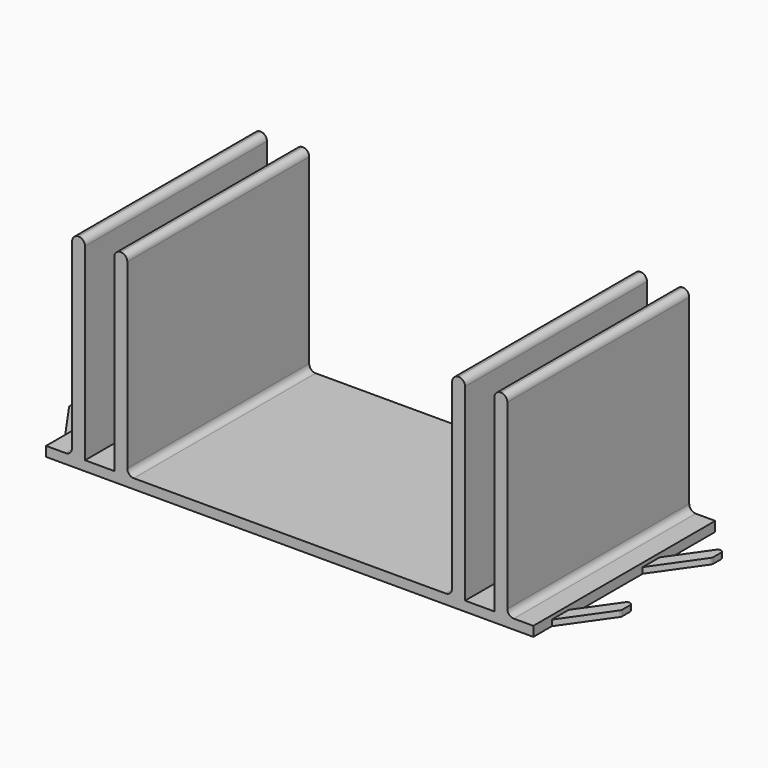
from build123d import *

# Parameters (mm, degrees)
F0_W     = 4
F0_H     = 60
F1_DEPTH = 70
F2_R     = 1.99999
F3_R     = 2
F5_DEPTH = 1.8
F6_R     = 1


# Not quite as in the source:
# - a fillet or chamfer is up to 0.001 mm smaller than in the source, because OpenCascade refuses the exact size


with BuildPart() as f1:
    # F0 (on Front) → F1 (new body)
    with BuildSketch(Plane.XZ):
        Polygon((0, -20), (0, -23), (65, -23), (65, -21), (67, -21), (67, -20), (63, -20), (54, -20), (50, -20), align=None)
        Polygon((-65, -23), (0, -23), (0, -20), (-50, -20), (-54, -20), (-63, -20), (-67, -20), (-67, -21), (-65, -21), align=None)
        Polygon((65, -21), (65, -23), (71, -23), (71, -22.25), (71, -21), (67, -21), align=None)
        Polygon((-71, -23), (-65, -23), (-65, -21), (-67, -21), (-71, -21), (-71, -22.25), align=None)
        Polygon((71, -22.25), (71, -23), (75, -23), (75, -21), (71, -21), align=None)
        with Locations((52, 10)):
            Rectangle(F0_W, F0_H)
        with Locations((-52, 10)):
            Rectangle(F0_W, F0_H)
        Polygon((-75, -23), (-71, -23), (-71, -22.25), (-71, -21), (-75, -21), align=None)
        Polygon((67, -20), (67, -21), (71, -21), (75, -21), (75, -20), align=None)
        Polygon((-71, -21), (-67, -21), (-67, -20), (-75, -20), (-75, -21), align=None)
        with Locations((65, 10)):
            Rectangle(F0_W, F0_H)
        with Locations((-65, 10)):
            Rectangle(F0_W, F0_H)
    extrude(amount=F1_DEPTH)

    # F2 (radius 2 in the source; OpenCascade refuses exactly that, so slightly less here)
    f2_edges = [f1.edges().sort_by_distance(p)[0] for p in [
        (-67, -35, 40),
        (-63, -35, 40),
        (-54, -35, 40),
        (-50, -35, 40),
        (54, -35, 40),
        (50, -35, 40),
        (63, -35, 40),
        (67, -35, 40),
    ]]
    fillet(f2_edges, radius=F2_R)

    # F3
    f3_edges = [f1.edges().sort_by_distance(p)[0] for p in [
        (-50, -35, -20),
        (50, -35, -20),
        (-67, -35, -20),
        (67, -35, -20),
    ]]
    fillet(f3_edges, radius=F3_R)

    # F4 (on face) → F5 (join)
    with BuildSketch(Plane(origin=(0, 0, -23), x_dir=(1, 0, 0), z_dir=(0, 0, -1))):
        Polygon((-85, 42.1), (-75, 56.3814800674), (-75, 62.9), (-85, 48.6185199326), align=None)
        Polygon((-75, 21.3814800674), (-75, 27.9), (-85, 13.6185199326), (-85, 7.1), align=None)
        Polygon((85, 13.6185199326), (75, 27.9), (75, 21.3814800674), (85, 7.1), align=None)
        Polygon((75, 62.9), (75, 56.3814800674), (85, 42.1), (85, 48.6185199326), align=None)
    extrude(amount=-F5_DEPTH)

    # F6
    f6_edges = [f1.edges().sort_by_distance(p)[0] for p in [
        (85, -42.1, -22.1),
        (85, -7.1, -22.1),
        (85, -13.61852, -22.1),
        (85, -48.61852, -22.1),
        (-85, -7.1, -22.1),
        (-85, -13.61852, -22.1),
        (-85, -42.1, -22.1),
        (-85, -48.61852, -22.1),
    ]]
    fillet(f6_edges, radius=F6_R)


solid = f1.part
